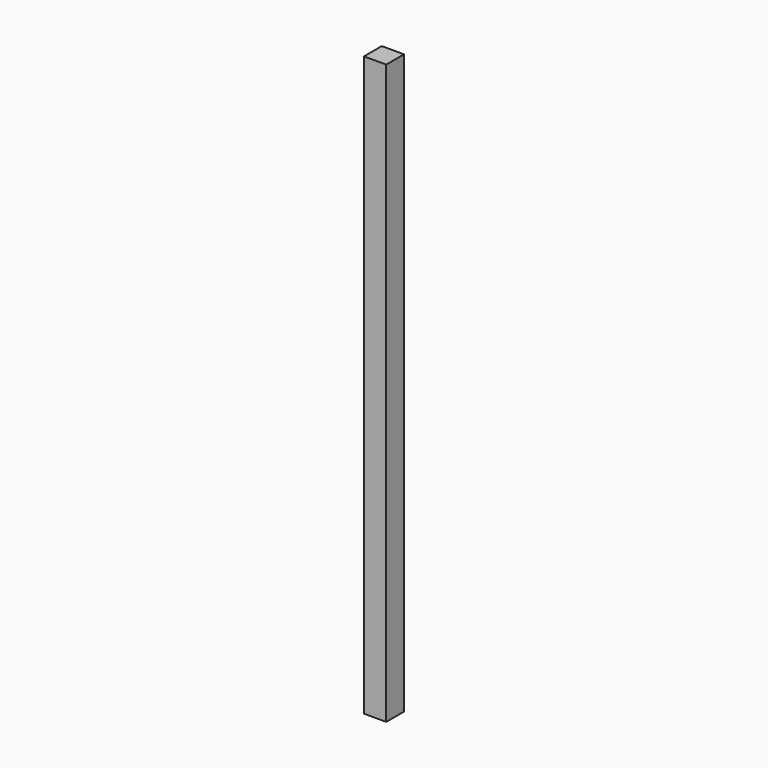
from build123d import *

# Parameters (mm, degrees)
F0_W     = 3.175
F0_H     = 82.55
F1_DEPTH = 3.175


# Not quite as in the source:
# - a feature names something its author has since deleted; it is built from what else it names


with BuildPart() as f1:
    # F0 (on Right) → F1 (new body)
    with BuildSketch(Plane.YZ):
        with Locations((1.5875, 41.275)):
            Rectangle(F0_W, F0_H)
    extrude(amount=F1_DEPTH)


solid = f1.part
